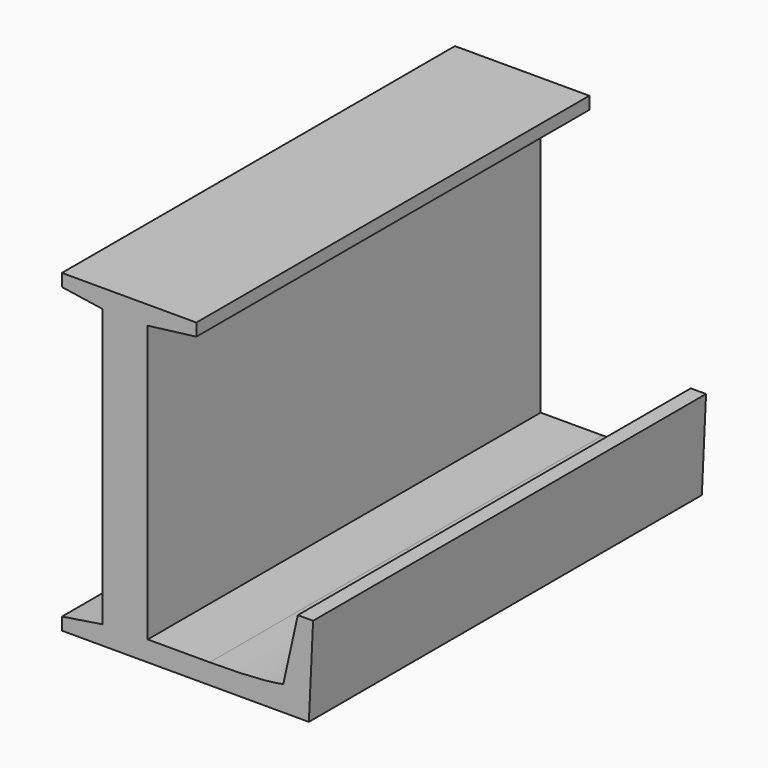
from build123d import *

# Parameters (mm, degrees)
F0_TEXT_SIZE = 74.6258935042
F1_DEPTH     = 38.1


# Not quite as in the source:
# - Text() gives the source's letters only with a copy of the font that has no kerning and outlines rounded to 1/6400 em; it was checked with that copy


with BuildPart() as f1:
    # F0 (on Front) → F1 (new body, symmetric)
    with BuildSketch(Plane.XZ):
        with Locations((-45.7666612506, 0)):
            Text('L', F0_TEXT_SIZE, font='Tinos', text_align=(TextAlign.LEFT, TextAlign.BOTTOM))
    extrude(amount=F1_DEPTH, both=True)


solid = f1.part
